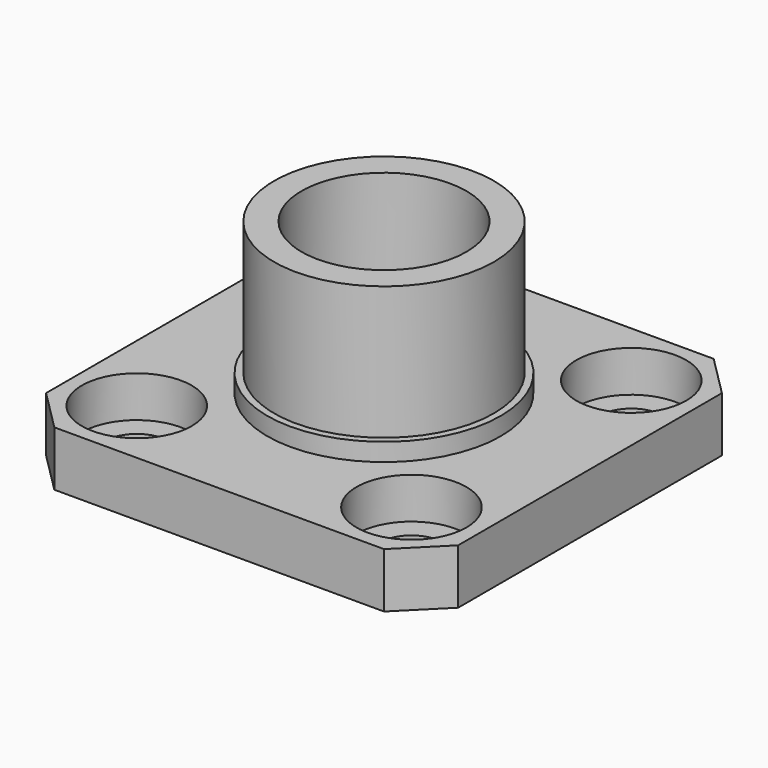
from build123d import *

# Parameters (mm, degrees)
F0_W     = 15
F0_H     = 15
F0_R     = 2
F0_R_2   = 4.25
F1_DEPTH = 2
F0_R_3   = 4
F2_DEPTH = 2.65
F0_R_4   = 3.7599999923
F0_R_5   = 3
F3_DEPTH = 7.5
F0_R_6   = 2.15
F4_DEPTH = 3.5
F5_DEPTH = 2.5
F6_SIZE  = 1.5
F0_R_7   = 1.15
F7_DEPTH = 0.5


with BuildPart() as f1:
    # F0 (on Top) → F1 (new body)
    with BuildSketch(Plane.XY):
        Rectangle(F0_W, F0_H)
        with Locations((-5, -5)):
            Circle(F0_R, mode=Mode.SUBTRACT)
        with Locations((5, -5)):
            Circle(F0_R, mode=Mode.SUBTRACT)
        with Locations((-5, 5)):
            Circle(F0_R, mode=Mode.SUBTRACT)
        Circle(F0_R_2, mode=Mode.SUBTRACT)
        with Locations((5, 5)):
            Circle(F0_R, mode=Mode.SUBTRACT)
    extrude(amount=F1_DEPTH)

    # F0 (on Top) → F2 (join)
    with BuildSketch(Plane.XY):
        Circle(F0_R_2)
        Circle(F0_R_3, mode=Mode.SUBTRACT)
    extrude(amount=F2_DEPTH)

    # F0 (on Top) → F3 (join)
    with BuildSketch(Plane.XY):
        Circle(F0_R_3)
        Circle(F0_R_4, mode=Mode.SUBTRACT)
        Circle(F0_R_4)
        Circle(F0_R_5, mode=Mode.SUBTRACT)
    extrude(amount=F3_DEPTH)

    # F0 (on Top) → F4 (join)
    with BuildSketch(Plane.XY):
        Circle(F0_R_4)
        Circle(F0_R_5, mode=Mode.SUBTRACT)
        Circle(F0_R_5)
        Circle(F0_R_6, mode=Mode.SUBTRACT)
    extrude(amount=F4_DEPTH)

    # F0 (on Top) → F5 (cut)
    with BuildSketch(Plane.XY):
        Circle(F0_R_5)
        Circle(F0_R_6, mode=Mode.SUBTRACT)
    extrude(amount=F5_DEPTH, mode=Mode.SUBTRACT)

    # F6
    f6_edges = [f1.edges().sort_by_distance(p)[0] for p in [
        (7.5, -7.5, 1),
        (7.5, 7.5, 1),
        (-7.5, -7.5, 1),
        (-7.5, 7.5, 1),
    ]]
    chamfer(f6_edges, length=F6_SIZE)

    # F0 (on Top) → F7 (join)
    with BuildSketch(Plane.XY):
        with Locations((-5, 5)):
            Circle(F0_R)
        with Locations((-5, 5)):
            Circle(F0_R_7, mode=Mode.SUBTRACT)
        with Locations((5, 5)):
            Circle(F0_R)
        with Locations((5, 5)):
            Circle(F0_R_7, mode=Mode.SUBTRACT)
        with Locations((5, -5)):
            Circle(F0_R)
        with Locations((5, -5)):
            Circle(F0_R_7, mode=Mode.SUBTRACT)
        with Locations((-5, -5)):
            Circle(F0_R)
        with Locations((-5, -5)):
            Circle(F0_R_7, mode=Mode.SUBTRACT)
    extrude(amount=F7_DEPTH)


solid = f1.part
